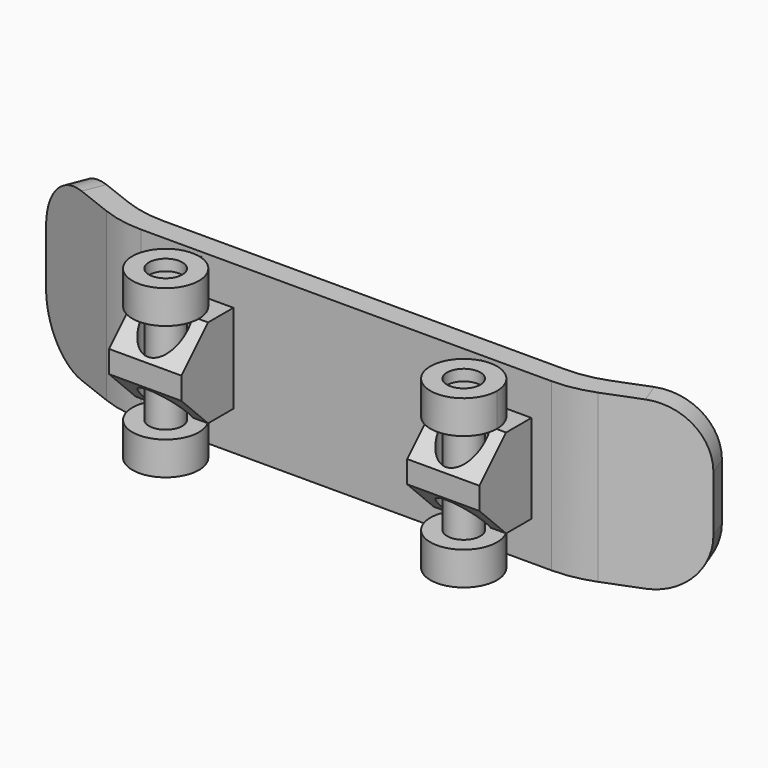
from build123d import *

# Parameters (mm, degrees)
F1_DEPTH    = 7.5
F2_R        = 5
F3_R        = 10
F4_W        = 6.5123213332
F4_H        = 5.8516720749
F4_R        = 2
F5_DEPTH    = 4
F4_R_2      = 1.5
F6_DEPTH    = 6.5
F7_T1_DEPTH = 21.942419261
F8_R        = 3
F8_R_2      = 1.5
F9_DEPTH    = 1
F10_DEPTH   = 1
F14_DEPTH   = 5


# Not quite as in the source:
# - a fillet or chamfer that OpenCascade refuses, or shapes differently, is made with other operations: its cross-section is extruded or revolved along the edge and cut away or added


with BuildPart() as f1:
    # F0 (on Top) → F1 (new body, symmetric)
    with BuildSketch(Plane.XY):
        Polygon((20, 0), (0, 0), (-20, 0), (-29.3166648167, 3.6331469407), (-30.0432942049, 1.7698139773), (-20.3761671049, -2), (0, -2), (20.3761671049, -2), (30.0432942049, 1.7698139773), (29.3166648167, 3.6331469407), align=None)
    extrude(amount=F1_DEPTH, both=True)

    # F2
    f2_edges = [f1.edges().sort_by_distance(p)[0] for p in [
        (29.67998, 2.70148, 7.5),
        (29.67998, 2.70148, -7.5),
        (-29.67998, 2.70148, 7.5),
        (-29.67998, 2.70148, -7.5),
    ]]
    fillet(f2_edges, radius=F2_R)

    # F3
    f3_edges = [f1.edges().sort_by_distance(p)[0] for p in [
        (20, 0, 0),
        (-20, 0, 0),
        (-20.376167, -2, 0),
        (20.376167, -2, 0),
    ]]
    fillet(f3_edges, radius=F3_R)

    # F4 (on Top) → F5 (join)
    with BuildSketch(Plane.XY):
        with Locations((13.4171620011, -4.9258360375)):
            Rectangle(F4_W, F4_H)
        with Locations((13.4171620011, -5.5516720749)):
            Circle(F4_R, mode=Mode.SUBTRACT)
    extrude(amount=F5_DEPTH)

    # F7: chamfer of 3 on 1 edges, made by hand

    # F7_s2 → F7_t1 (cut)
    with BuildSketch(Plane.YZ.offset(2.4459523706)):
        Polygon((-4.8516720749, 4), (-7.8516720749, 1), (-7.8516720749, 4), align=None)
    extrude(amount=F7_T1_DEPTH, mode=Mode.SUBTRACT)


with BuildPart() as f6:
    # F4 (on Top) → F6 (new body, symmetric)
    with BuildSketch(Plane.XY):
        with Locations((13.4171620011, -5.5516720749)):
            Circle(F4_R_2)
    extrude(amount=F6_DEPTH, both=True)

    # F8 (on face) → F9 (join, symmetric)
    with BuildSketch(Plane.XY.offset(6.5)):
        with Locations((13.4171620011, -5.5516720749)):
            Circle(F8_R)
        with Locations((13.4171620011, -5.5516720749)):
            Circle(F8_R_2, mode=Mode.SUBTRACT)
    extrude(amount=F9_DEPTH, both=True)

    # F10 (add): a face of the model
    f10_faces = [f6.faces().sort_by_distance(p)[0] for p in [
        (10.5020148149, -5.5516720749, 5.5),
    ]]
    extrude(f10_faces, amount=F10_DEPTH)


with BuildPart() as f11_1:
    # F11: instance of F1
    add(f1.part.mirror(Plane.XY))


with BuildPart() as f11_2:
    # F11: instance of F6
    add(f6.part.mirror(Plane.XY))


with BuildPart() as f1_1:
    add(f1.part)

    add(f11_1.part)  # F12 merges F11_1
    # F12: F11_2, F11_1, F6, F1 across plane
    add(f11_2.part.mirror(Plane.YZ))
    add(f11_1.part.mirror(Plane.YZ))
    add(f6.part.mirror(Plane.YZ))
    add(f1.part.mirror(Plane.YZ))

    add(f6.part)  # F14 merges F6
    # F13 (on face) → F14 (join)
    with BuildSketch(Plane.XY.offset(7.5)):
        with BuildLine():
            Line((12.6132123219, -2.5642015695), (12.6032123219, -2.5642015695))
            Line((12.6032123219, -2.5642015695), (12.6032123219, -2.6642015695))
            ThreePointArc((12.6032123219, -2.6642015695), (12.6082111102, -2.6627971285), (12.6132123219, -2.6614013414))
            Line((12.6132123219, -2.6614013414), (12.6132123219, -2.5642015695))
        make_face()
    extrude(amount=-F14_DEPTH)



with BuildPart() as f1_2:
    add(f1_1.part)

    add(f11_2.part)  # F15 merges F11_2
    # F15: F1 across plane
    add(f1_1.part.mirror(Plane.YZ))

    # F16: union 


solid = f1_2.part
